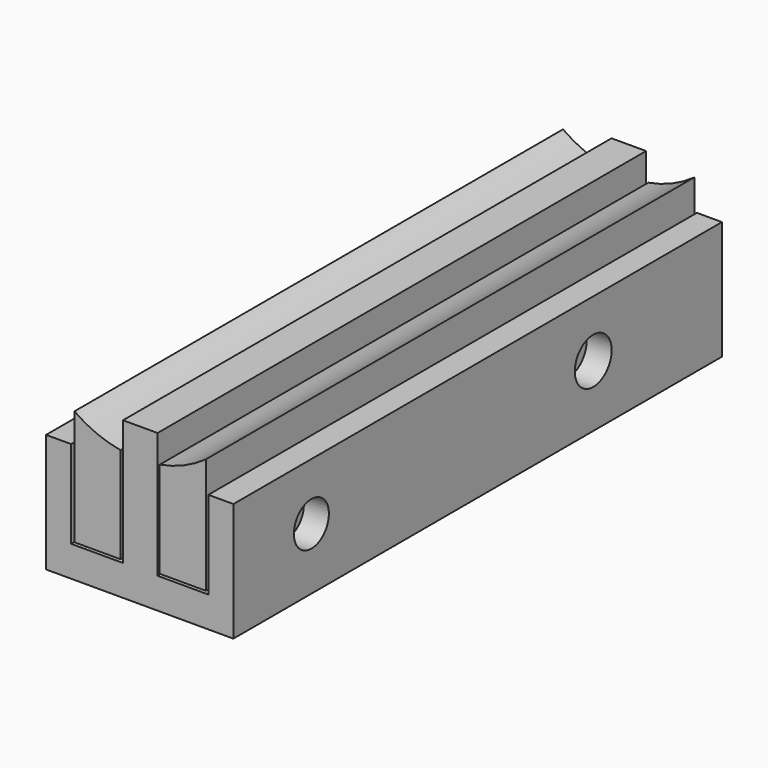
from build123d import *

# Parameters (mm, degrees)
F1_W     = 3.2777013257
F1_H     = 11.5029346198
F1_W_2   = 4.52345144
F1_H_2   = 4.1451063007
F1_H_3   = 16.4643982425
F2_DEPTH = 80
F5_R     = 3.0180179705
F5_R_2   = 2.8661340768
F6_DEPTH = 77
F7_DEPTH = 9
F8_DEPTH = 8


with BuildPart() as f2:
    # F1 (on Front) → F2 (new body)
    with BuildSketch(Plane.XZ):
        with Locations((10.6315002777, -21.6521834955)):
            Rectangle(F1_W, F1_H)
        with Locations((-10.6315002777, -21.6521834955)):
            Rectangle(F1_W, F1_H)
        with Locations((0.0701001845, -29.4762039557)):
            Rectangle(F1_W_2, F1_H_2)
        with Locations((0.0701001845, -19.1714516841)):
            Rectangle(F1_W_2, F1_H_3)
        Polygon((-2.1916255355, -31.5487571061), (-2.1916255355, -27.4036508054), (-8.9926496148, -27.4036508054), (-12.2703509405, -27.4036508054), (-12.2703509405, -39.4294504076), (12.2703509405, -39.4294504076), (12.2703509405, -27.4036508054), (8.9926496148, -27.4036508054), (2.3318259045, -27.4036508054), (2.3318259045, -31.5487571061), align=None)
    extrude(amount=F2_DEPTH)

    # F5 (on face) → F6 (cut)
    with BuildSketch(Plane(origin=(-12.2703509405, 0, 0), x_dir=(0, -1, 0), z_dir=(-1, 0, 0))):
        with Locations((21.0752002895, -23.3381781727)):
            Circle(F5_R)
        with Locations((67.2274827957, -23.3729947358)):
            Circle(F5_R_2)
    extrude(amount=-F6_DEPTH, mode=Mode.SUBTRACT)

    # F7 (add): a face of the model
    f7_faces = [f2.faces().sort_by_distance(p)[0] for p in [
        (0, -40, -39.4294504076),
    ]]
    extrude(f7_faces, amount=-F7_DEPTH)

    # F8 (cut): a face of the model
    f8_faces = [f2.faces().sort_by_distance(p)[0] for p in [
        (0, -40, -39.4294504076),
    ]]
    extrude(f8_faces, amount=-F8_DEPTH, mode=Mode.SUBTRACT)


with BuildPart() as f2b:
    # F0 (on Front) → F2, piece 2 (new body)
    with BuildSketch(Plane.XZ):
        with BuildLine():
            Line((8.6488667876, -27.0813219249), (8.6488667876, -11.9249372814))
            ThreePointArc((8.6488667876, -11.9249372814), (5.7787876042, -13.5503741535), (2.6189955003, -14.4964784842))
            Line((2.6189955003, -14.4964784842), (2.6189955003, -27.0813219249))
            Line((2.6189955003, -27.0813219249), (8.6488667876, -27.0813219249))
        make_face()
    extrude(amount=F2_DEPTH)


with BuildPart() as f2c:
    # F0 (on Front) → F2, piece 3 (new body)
    with BuildSketch(Plane.XZ):
        with BuildLine():
            ThreePointArc((-2.5203907914, -14.4964784842), (-5.6771197832, -13.5746296138), (-8.5502620786, -11.9746931723))
            Line((-8.5502620786, -11.9746931723), (-8.5502620786, -27.0813219249))
            Line((-8.5502620786, -27.0813219249), (-2.5203907914, -27.0813219249))
            Line((-2.5203907914, -27.0813219249), (-2.5203907914, -14.4964784842))
        make_face()
    extrude(amount=F2_DEPTH)


solid = Compound([f2.part, f2b.part, f2c.part])
